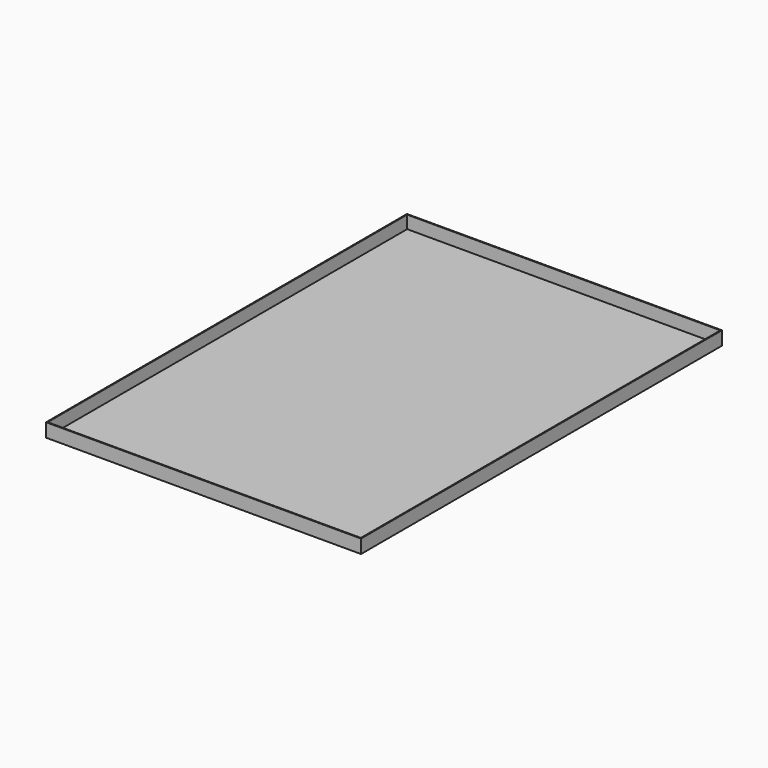
from build123d import *

# Parameters (mm, degrees)
F0_W     = 1168.4
F0_H     = 1676.4
F1_DEPTH = 3.175
F2_W     = 1168.4
F2_H     = 3.175
F3_DEPTH = 50.8


# Not quite as in the source:
# - a length typed as a fraction of an inch, garbled in the dataset ("3 / 203.2 mm" for 3/8 in), is restored


with BuildPart() as f1:
    # F0 (on Top) → F1 (new body)
    with BuildSketch(Plane.XY):
        with Locations((-584.2, 838.2)):
            Rectangle(F0_W, F0_H)
    extrude(amount=F1_DEPTH)

    # F2 (on Top) → F3 (join)
    with BuildSketch(Plane.XY):
        Polygon((-1168.4, -3.175), (-1168.4, 0), (-1168.4, 1676.4), (-1168.4, 1679.575), (-1171.575, 1679.575), (-1171.575, -3.175), align=None)
        with Locations((-584.2, 1677.9875)):
            Rectangle(F2_W, F2_H)
        Polygon((0, 1676.4), (0, 0), (0, -3.175), (3.175, -3.175), (3.175, 1679.575), (0, 1679.575), align=None)
        with Locations((-584.2, -1.5875)):
            Rectangle(F2_W, F2_H)
    extrude(amount=F3_DEPTH)


solid = f1.part
